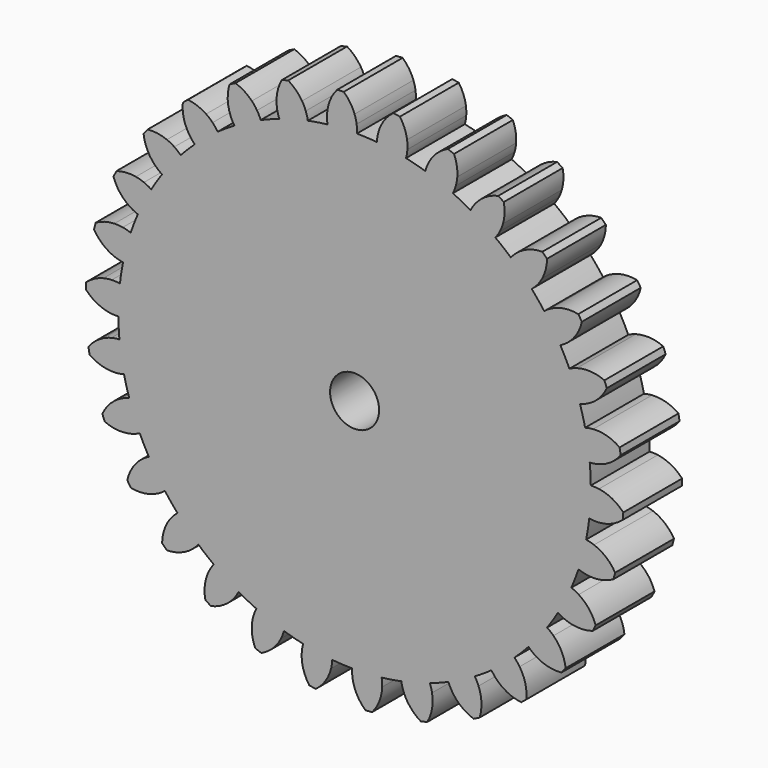
from build123d import *

# Parameters (mm, degrees)
F0_R            = 3.175
F1_DEPTH        = 9.525
F1_COPIES_COUNT = 30


# Not quite as in the source:
# - a feature of the source that left no trace in its solid (it failed there, or was rolled back) is left out
# - a pattern or mirror of a feature is missing from the dataset's text; its kind, count and spacing are read off the source's solid


with BuildPart() as f1:
    # F0 (on Front) → F1 (new body)
    with BuildSketch(Plane.XZ):
        with BuildLine():
            ThreePointArc((-3.5055472024, 30.3860761508), (-20.3516109929, -22.8345005425), (30.5876198, 0))
            ThreePointArc((30.5876198, 0), (21.7380856307, 21.5187852385), (0.3101336033, 30.5860475083))
            ThreePointArc((0.3101336033, 30.5860475083), (-1.6008323314, 30.5457005301), (-3.5055472024, 30.3860761508))
        make_face()
        Circle(F0_R, mode=Mode.SUBTRACT)
        with BuildLine():
            ThreePointArc((-3.5055472024, 30.3860761508), (-1.6008323314, 30.5457005301), (0.3101336033, 30.5860475083))
            ThreePointArc((0.3101336033, 30.5860475083), (0.3144620421, 31.1165571034), (0.2656482324, 31.6448339038))
            ThreePointArc((0.2656482324, 31.6448339038), (0.1602319802, 32.181428283), (0, 32.704278))
            ThreePointArc((0, 32.704278), (-0.5715118632, 33.8325647691), (-1.3944415291, 34.7930040477))
            ThreePointArc((-1.3944415291, 34.7930040477), (-1.8223869933, 34.7732153171), (-2.250056613, 34.7481631613))
            ThreePointArc((-2.250056613, 34.7481631613), (-3.1971627604, 33.2104080788), (-3.5719788419, 31.4437123911))
            ThreePointArc((-3.5719788419, 31.4437123911), (-3.5653052823, 30.9132271138), (-3.5055472024, 30.3860761508))
        make_face()
    extrude(amount=F1_DEPTH)

    # F1_copies: F1 ×30 about axis
    f1_copies_axis = Axis((0, 0, 0), (0, 1, 0))


with BuildPart() as f1_1:
    add(f1.part)
    for i in range(1, F1_COPIES_COUNT):
        add(f1.part.rotate(f1_copies_axis, i * 360 / F1_COPIES_COUNT))


solid = f1_1.part
